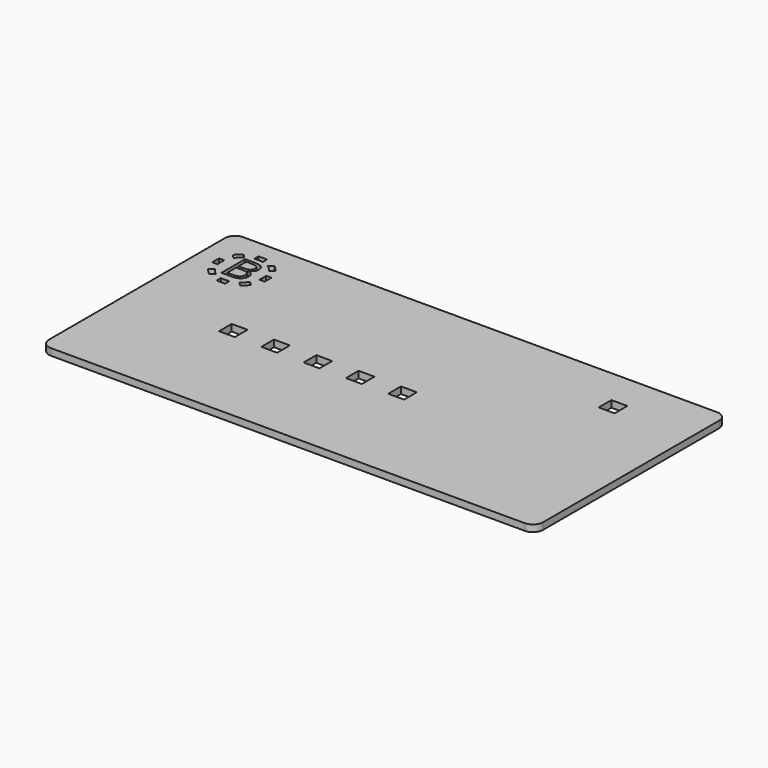
from build123d import *

# Parameters (mm, degrees)
F1_DEPTH     = 2.032
F2_TEXT_SIZE = 12.4457473349
F3_DEPTH     = 2.032
F4_W         = 4.7625
F4_H         = 4.7625
F4_W_2       = 4.7752
F4_H_2       = 4.7752
F5_DEPTH     = 2.032


# Not quite as in the source:
# - Text() gives the source's letters only with a copy of the font that has no kerning and outlines rounded to 1/6400 em; it was checked with that copy


with BuildPart() as f1:
    # F0 (on Top) → F1 (new body)
    with BuildSketch(Plane.XY):
        with BuildLine():
            Line((3.048, 0), (0, 0))
            Line((0, 0), (0, 3.048))
            Line((0, 3.048), (-142.24, 3.048))
            ThreePointArc((-142.24, 3.048), (-144.3952614691, 2.1552614691), (-145.288, 0))
            Line((-145.288, 0), (-145.288, -66.04))
            ThreePointArc((-145.288, -66.04), (-144.3952614691, -68.1952614691), (-142.24, -69.088))
            Line((-142.24, -69.088), (0, -69.088))
            ThreePointArc((0, -69.088), (2.1552614691, -68.1952614691), (3.048, -66.04))
            Line((3.048, -66.04), (3.048, -33.02))
            Line((3.048, -33.02), (3.048, 0))
        make_face()
        with BuildLine():
            Line((0, 3.048), (0, 0))
            Line((0, 0), (3.048, 0))
            ThreePointArc((3.048, 0), (2.1552614691, 2.1552614691), (0, 3.048))
        make_face()
    extrude(amount=F1_DEPTH)

    # F2 (on face) → F3 (cut)
    with BuildSketch(Plane.XY.offset(2.032)):
        with BuildLine():
            ThreePointArc((-137.3774346633, -6.6586165609), (-136.5701280605, -5.6698719395), (-135.5813834391, -4.8625653367))
            Line((-135.5813834391, -4.8625653367), (-136.749733183, -3.6942155928))
            Line((-136.749733183, -3.6942155928), (-137.6477587951, -4.5922412049))
            Line((-137.6477587951, -4.5922412049), (-138.5457844072, -5.490266817))
            Line((-138.5457844072, -5.490266817), (-137.3774346633, -6.6586165609))
        make_face()
        with BuildLine():
            ThreePointArc((-132.08, -3.81), (-131.4417680913, -3.8421554284), (-130.81, -3.9382960533))
            Line((-130.81, -3.9382960533), (-130.81, -2.286))
            Line((-130.81, -2.286), (-132.08, -2.286))
            Line((-132.08, -2.286), (-132.08, -3.81))
        make_face()
        with BuildLine():
            ThreePointArc((-133.35, -3.9382960533), (-132.7182319087, -3.8421554284), (-132.08, -3.81))
            Line((-132.08, -3.81), (-132.08, -2.286))
            Line((-132.08, -2.286), (-133.35, -2.286))
            Line((-133.35, -2.286), (-133.35, -3.9382960533))
        make_face()
        with BuildLine():
            ThreePointArc((-128.5786165609, -4.8625653367), (-127.5898719395, -5.6698719395), (-126.7825653367, -6.6586165609))
            Line((-126.7825653367, -6.6586165609), (-125.6142155928, -5.490266817))
            Line((-125.6142155928, -5.490266817), (-126.5122412049, -4.5922412049))
            Line((-126.5122412049, -4.5922412049), (-127.410266817, -3.6942155928))
            Line((-127.410266817, -3.6942155928), (-128.5786165609, -4.8625653367))
        make_face()
        with BuildLine():
            ThreePointArc((-125.8582960533, -8.89), (-125.7621554284, -9.5217680913), (-125.73, -10.16))
            ThreePointArc((-125.73, -10.16), (-125.7621554284, -10.7982319087), (-125.8582960533, -11.43))
            Line((-125.8582960533, -11.43), (-124.206, -11.43))
            Line((-124.206, -11.43), (-124.206, -10.16))
            Line((-124.206, -10.16), (-124.206, -8.89))
            Line((-124.206, -8.89), (-125.8582960533, -8.89))
        make_face()
        with BuildLine():
            Line((-125.6142155928, -14.829733183), (-126.7825653367, -13.6613834391))
            ThreePointArc((-126.7825653367, -13.6613834391), (-127.5898719395, -14.6501280605), (-128.5786165609, -15.4574346633))
            Line((-128.5786165609, -15.4574346633), (-127.410266817, -16.6257844072))
            Line((-127.410266817, -16.6257844072), (-126.5122412049, -15.7277587951))
            Line((-126.5122412049, -15.7277587951), (-125.6142155928, -14.829733183))
        make_face()
        with BuildLine():
            Line((-130.81, -18.034), (-130.81, -16.3817039467))
            ThreePointArc((-130.81, -16.3817039467), (-132.08, -16.51), (-133.35, -16.3817039467))
            Line((-133.35, -16.3817039467), (-133.35, -18.034))
            Line((-133.35, -18.034), (-132.08, -18.034))
            Line((-132.08, -18.034), (-130.81, -18.034))
        make_face()
        with BuildLine():
            Line((-136.749733183, -16.6257844072), (-135.5813834391, -15.4574346633))
            ThreePointArc((-135.5813834391, -15.4574346633), (-136.5701280605, -14.6501280605), (-137.3774346633, -13.6613834391))
            Line((-137.3774346633, -13.6613834391), (-138.5457844072, -14.829733183))
            Line((-138.5457844072, -14.829733183), (-137.6477587951, -15.7277587951))
            Line((-137.6477587951, -15.7277587951), (-136.749733183, -16.6257844072))
        make_face()
        with BuildLine():
            Line((-139.954, -11.43), (-138.3017039467, -11.43))
            ThreePointArc((-138.3017039467, -11.43), (-138.43, -10.16), (-138.3017039467, -8.89))
            Line((-138.3017039467, -8.89), (-139.954, -8.89))
            Line((-139.954, -8.89), (-139.954, -10.16))
            Line((-139.954, -10.16), (-139.954, -11.43))
        make_face()
        with Locations((-136.1339241266, -14.2642897554)):
            Text('B', F2_TEXT_SIZE, font='Open Sans', text_align=(TextAlign.LEFT, TextAlign.BOTTOM))
    extrude(amount=-F3_DEPTH, mode=Mode.SUBTRACT)

    # F4 (on face) → F5 (cut)
    with BuildSketch(Plane.XY.offset(2.032)):
        with Locations((-114.45875, -35.40125)):
            Rectangle(F4_W, F4_H)
        with Locations((-101.75875, -35.40125)):
            Rectangle(F4_W, F4_H)
        with Locations((-89.05875, -35.40125)):
            Rectangle(F4_W, F4_H)
        with Locations((-76.35875, -35.40125)):
            Rectangle(F4_W, F4_H)
        with Locations((-63.65875, -35.40125)):
            Rectangle(F4_W, F4_H)
        with Locations((-20.7899, -10.0076)):
            Rectangle(F4_W_2, F4_H_2)
    extrude(amount=-F5_DEPTH, mode=Mode.SUBTRACT)


solid = f1.part
